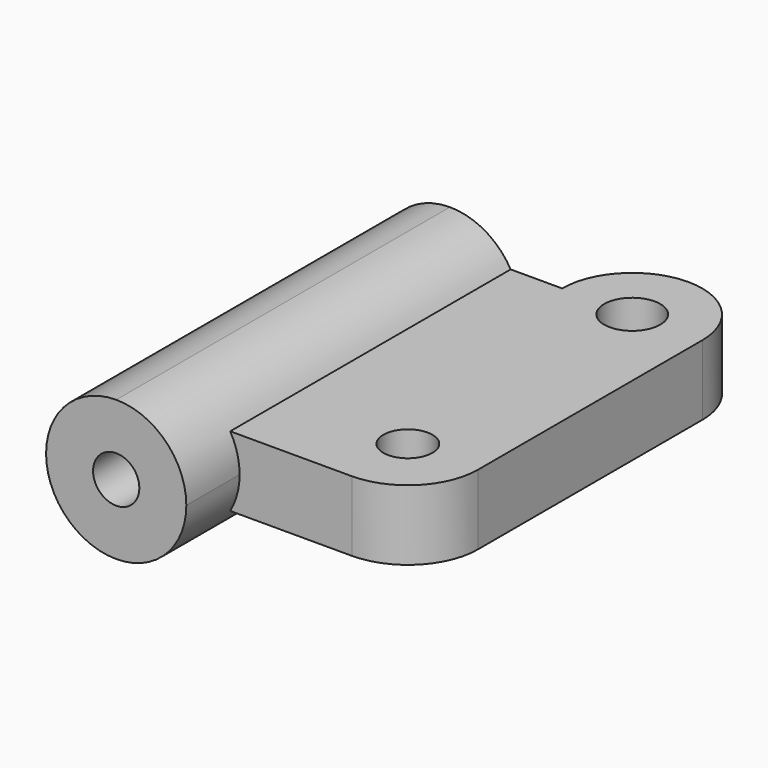
from build123d import *

# Parameters (mm, degrees)
F0_R     = 1.75
F0_R_2   = 2
F1_DEPTH = 5
F2_DEPTH = 7.5
F3_DEPTH = 2.5
F4_R     = 1.65
F5_DEPTH = 29.75
F6_R     = 4.99999


# Not quite as in the source:
# - a fillet or chamfer is up to 0.001 mm smaller than in the source, because OpenCascade refuses the exact size


with BuildPart() as f1:
    # F0 (on Top) → F1 (new body)
    with BuildSketch(Plane.XY):
        with BuildLine():
            Line((-5, 10), (-8, 10))
            Line((-8, 10), (-8, -15))
            Line((-8, -15), (0, -15))
            ThreePointArc((0, -15), (3.5355339059, -13.5355339059), (5, -10))
            Line((5, -10), (5, 10))
            ThreePointArc((5, 10), (0, 15), (-5, 10))
        make_face()
        with Locations((0, -10)):
            Circle(F0_R, mode=Mode.SUBTRACT)
        with Locations((0, 10)):
            Circle(F0_R_2, mode=Mode.SUBTRACT)
    extrude(amount=F1_DEPTH)

    # F0 (on Top) → F2 (join)
    with BuildSketch(Plane.XY):
        Polygon((-8, 10), (-18, 10), (-18, -19.75), (-8, -19.75), (-8, -15), align=None)
    extrude(amount=F2_DEPTH)

    # F0 (on Top) → F3 (join)
    with BuildSketch(Plane.XY):
        Polygon((-8, 10), (-18, 10), (-18, -19.75), (-8, -19.75), (-8, -15), align=None)
    extrude(amount=-F3_DEPTH)

    # F4 (on face) → F5 (cut, through all)
    with BuildSketch(Plane.XZ.offset(19.75)):
        with Locations((-13, 2.5)):
            Circle(F4_R)
    extrude(amount=-F5_DEPTH, mode=Mode.SUBTRACT)

    # F6 (radius 5 in the source; OpenCascade refuses exactly that, so slightly less here)
    f6_edges = [f1.edges().sort_by_distance(p)[0] for p in [
        (-18, -4.875, 7.5),
        (-18, -4.875, -2.5),
        (-8, -4.875, 7.5),
        (-8, -4.875, -2.5),
    ]]
    fillet(f6_edges, radius=F6_R)


solid = f1.part
